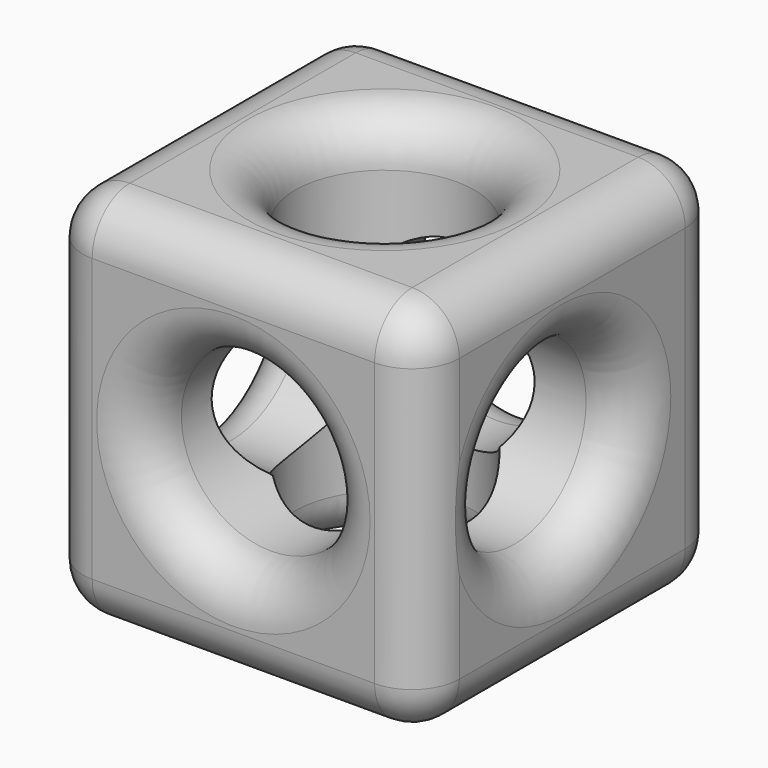
from build123d import *

# Parameters (mm, degrees)
F0_W         = 50.8
F0_H         = 50.8
F1_DEPTH     = 50.8
F3_D         = 24.20874
F5_D         = 24.20874
F7_D         = 24.20874
F8_T1_DEPTH  = 38.1
F8_T3_DEPTH  = 38.1
F8_T5_DEPTH  = 38.1
F8_S9_W      = 6.35
F8_S9_H      = 6.35
F8_T10_DEPTH = 6.35
F8_S15_W     = 6.35
F8_S15_H     = 6.35
F8_T16_DEPTH = 6.35
F8_S21_W     = 6.35
F8_S21_H     = 6.35
F8_T22_DEPTH = 6.35
F8_S27_W     = 6.35
F8_S27_H     = 6.35
F8_T28_DEPTH = 6.35
F8_S33_W     = 6.35
F8_S33_H     = 6.35
F8_T34_DEPTH = 6.35
F8_S39_W     = 6.35
F8_S39_H     = 6.35
F8_T40_DEPTH = 6.35
F8_S45_W     = 6.35
F8_S45_H     = 6.35
F8_T46_DEPTH = 6.35
F8_S51_W     = 6.35
F8_S51_H     = 6.35
F8_T52_DEPTH = 6.35


# Not quite as in the source:
# - a fillet or chamfer that OpenCascade refuses, or shapes differently, is made with other operations: its cross-section is extruded or revolved along the edge and cut away or added


with BuildPart() as f1:
    # F0 (on Front) → F1 (new body)
    with BuildSketch(Plane.XZ):
        Rectangle(F0_W, F0_H)
    extrude(amount=F1_DEPTH)

    # F3 (through all)
    with Locations(Plane.XZ.offset(50.8)):
        with Locations((0, 0)):
            Hole(F3_D / 2)

    # F5 (through all)
    with Locations(Plane.XY.offset(25.4)):
        with Locations((0, -25.266315788)):
            Hole(F5_D / 2)

    # F7 (through all)
    with Locations(Plane.YZ.offset(25.4)):
        with Locations((-27.2314734757, 0)):
            Hole(F7_D / 2)

    # F8: fillet of radius 6.35 on 18 edges, made by hand

    # F8_s2 → F8_t1 (cut)
    with BuildSketch(Plane.YZ.offset(-19.05)):
        with BuildLine():
            ThreePointArc((-50.8, 19.05), (-48.9401280605, 23.5401280605), (-44.45, 25.4))
            Line((-44.45, 25.4), (-50.8, 25.4))
            Line((-50.8, 25.4), (-50.8, 19.05))
        make_face()
        with BuildLine():
            ThreePointArc((0, 19.05), (-1.8598719395, 23.5401280605), (-6.35, 25.4))
            Line((-6.35, 25.4), (0, 25.4))
            Line((0, 25.4), (0, 19.05))
        make_face()
        with BuildLine():
            ThreePointArc((-44.45, -25.4), (-48.9401280605, -23.5401280605), (-50.8, -19.05))
            Line((-50.8, -19.05), (-50.8, -25.4))
            Line((-50.8, -25.4), (-44.45, -25.4))
        make_face()
        with BuildLine():
            ThreePointArc((-6.35, -25.4), (-1.8598719395, -23.5401280605), (0, -19.05))
            Line((0, -19.05), (0, -25.4))
            Line((0, -25.4), (-6.35, -25.4))
        make_face()
    extrude(amount=F8_T1_DEPTH, mode=Mode.SUBTRACT)

    # F8_s4 → F8_t3 (cut)
    with BuildSketch(Plane.XZ.offset(6.35)):
        with BuildLine():
            ThreePointArc((25.4, 19.05), (23.5401280605, 23.5401280605), (19.05, 25.4))
            Line((19.05, 25.4), (25.4, 25.4))
            Line((25.4, 25.4), (25.4, 19.05))
        make_face()
        with BuildLine():
            ThreePointArc((25.4, -19.05), (23.5401280605, -23.5401280605), (19.05, -25.4))
            Line((19.05, -25.4), (25.4, -25.4))
            Line((25.4, -25.4), (25.4, -19.05))
        make_face()
        with BuildLine():
            ThreePointArc((-19.05, 25.4), (-23.5401280605, 23.5401280605), (-25.4, 19.05))
            Line((-25.4, 19.05), (-25.4, 25.4))
            Line((-25.4, 25.4), (-19.05, 25.4))
        make_face()
        with BuildLine():
            ThreePointArc((-19.05, -25.4), (-23.5401280605, -23.5401280605), (-25.4, -19.05))
            Line((-25.4, -19.05), (-25.4, -25.4))
            Line((-25.4, -25.4), (-19.05, -25.4))
        make_face()
    extrude(amount=F8_T3_DEPTH, mode=Mode.SUBTRACT)

    # F8_s6 → F8_t5 (cut)
    with BuildSketch(Plane.XY.offset(-19.05)):
        with BuildLine():
            ThreePointArc((25.4, -44.45), (23.5401280605, -48.9401280605), (19.05, -50.8))
            Line((19.05, -50.8), (25.4, -50.8))
            Line((25.4, -50.8), (25.4, -44.45))
        make_face()
        with BuildLine():
            ThreePointArc((25.4, -6.35), (23.5401280605, -1.8598719395), (19.05, 0))
            Line((19.05, 0), (25.4, 0))
            Line((25.4, 0), (25.4, -6.35))
        make_face()
        with BuildLine():
            ThreePointArc((-19.05, -50.8), (-23.5401280605, -48.9401280605), (-25.4, -44.45))
            Line((-25.4, -44.45), (-25.4, -50.8))
            Line((-25.4, -50.8), (-19.05, -50.8))
        make_face()
        with BuildLine():
            ThreePointArc((-19.05, 0), (-23.5401280605, -1.8598719395), (-25.4, -6.35))
            Line((-25.4, -6.35), (-25.4, 0))
            Line((-25.4, 0), (-19.05, 0))
        make_face()
    extrude(amount=F8_T5_DEPTH, mode=Mode.SUBTRACT)


with BuildPart() as f8_tool8:
    # F8_s9 → F8_t10 (new body)
    with BuildSketch(Plane.YZ.offset(19.05)):
        with Locations((-47.625, 22.225)):
            Rectangle(F8_S9_W, F8_S9_H)
    extrude(amount=F8_T10_DEPTH)

    # F8_s11 → F8_t12 (revolve, cut)
    with BuildSketch(Plane(origin=(19.05, -44.45, 19.05), x_dir=(0, 0.7071067812, -0.7071067812), z_dir=(0, -0.7071067812, -0.7071067812))):
        with BuildLine():
            ThreePointArc((0, -6.35), (6.35, 0), (0, 6.35))
            Line((0, 6.35), (0, -6.35))
        make_face()
    revolve(axis=Axis((19.05, -44.45, 19.05), (1, 0, 0)), mode=Mode.SUBTRACT)


with BuildPart() as f1_1:
    add(f1.part)

    # F8_t7: cut F8_tool8
    add(f8_tool8.part, mode=Mode.SUBTRACT)


with BuildPart() as f8_tool14:
    # F8_s15 → F8_t16 (new body)
    with BuildSketch(Plane.XZ.offset(44.45)):
        with Locations((-22.225, 22.225)):
            Rectangle(F8_S15_W, F8_S15_H)
    extrude(amount=F8_T16_DEPTH)

    # F8_s17 → F8_t18 (revolve, cut)
    with BuildSketch(Plane(origin=(-19.05, -44.45, 19.05), x_dir=(0.7071067812, 0, -0.7071067812), z_dir=(-0.7071067812, 0, -0.7071067812))):
        with BuildLine():
            ThreePointArc((0, -6.35), (6.35, 0), (0, 6.35))
            Line((0, 6.35), (0, -6.35))
        make_face()
    revolve(axis=Axis((-19.05, -44.45, 19.05), (0, -1, 0)), mode=Mode.SUBTRACT)


with BuildPart() as f1_2:
    add(f1_1.part)

    # F8_t13: cut F8_tool14
    add(f8_tool14.part, mode=Mode.SUBTRACT)


with BuildPart() as f8_tool20:
    # F8_s21 → F8_t22 (new body)
    with BuildSketch(Plane.YZ.offset(19.05)):
        with Locations((-3.175, 22.225)):
            Rectangle(F8_S21_W, F8_S21_H)
    extrude(amount=F8_T22_DEPTH)

    # F8_s23 → F8_t24 (revolve, cut)
    with BuildSketch(Plane(origin=(19.05, -6.35, 19.05), x_dir=(0, -0.7071067812, -0.7071067812), z_dir=(0, -0.7071067812, 0.7071067812))):
        with BuildLine():
            ThreePointArc((0, -6.35), (6.35, 0), (0, 6.35))
            Line((0, 6.35), (0, -6.35))
        make_face()
    revolve(axis=Axis((19.05, -6.35, 19.05), (1, 0, 0)), mode=Mode.SUBTRACT)


with BuildPart() as f1_3:
    add(f1_2.part)

    # F8_t19: cut F8_tool20
    add(f8_tool20.part, mode=Mode.SUBTRACT)


with BuildPart() as f8_tool26:
    # F8_s27 → F8_t28 (new body)
    with BuildSketch(Plane.YZ.offset(19.05)):
        with Locations((-47.625, -22.225)):
            Rectangle(F8_S27_W, F8_S27_H)
    extrude(amount=F8_T28_DEPTH)

    # F8_s29 → F8_t30 (revolve, cut)
    with BuildSketch(Plane(origin=(19.05, -44.45, -19.05), x_dir=(0, 0.7071067812, 0.7071067812), z_dir=(0, 0.7071067812, -0.7071067812))):
        with BuildLine():
            ThreePointArc((0, -6.35), (6.35, 0), (0, 6.35))
            Line((0, 6.35), (0, -6.35))
        make_face()
    revolve(axis=Axis((19.05, -44.45, -19.05), (1, 0, 0)), mode=Mode.SUBTRACT)


with BuildPart() as f1_4:
    add(f1_3.part)

    # F8_t25: cut F8_tool26
    add(f8_tool26.part, mode=Mode.SUBTRACT)


with BuildPart() as f8_tool32:
    # F8_s33 → F8_t34 (new body)
    with BuildSketch(Plane.YZ.offset(19.05)):
        with Locations((-3.175, -22.225)):
            Rectangle(F8_S33_W, F8_S33_H)
    extrude(amount=F8_T34_DEPTH)

    # F8_s35 → F8_t36 (revolve, cut)
    with BuildSketch(Plane(origin=(19.05, -6.35, -19.05), x_dir=(0, -0.7071067812, 0.7071067812), z_dir=(0, 0.7071067812, 0.7071067812))):
        with BuildLine():
            ThreePointArc((0, -6.35), (6.35, 0), (0, 6.35))
            Line((0, 6.35), (0, -6.35))
        make_face()
    revolve(axis=Axis((19.05, -6.35, -19.05), (1, 0, 0)), mode=Mode.SUBTRACT)


with BuildPart() as f1_5:
    add(f1_4.part)

    # F8_t31: cut F8_tool32
    add(f8_tool32.part, mode=Mode.SUBTRACT)


with BuildPart() as f8_tool38:
    # F8_s39 → F8_t40 (new body)
    with BuildSketch(Plane.XZ.offset(6.35)):
        with Locations((-22.225, 22.225)):
            Rectangle(F8_S39_W, F8_S39_H)
    extrude(amount=-F8_T40_DEPTH)

    # F8_s41 → F8_t42 (revolve, cut)
    with BuildSketch(Plane(origin=(-19.05, -6.35, 19.05), x_dir=(0.7071067812, 0, -0.7071067812), z_dir=(0.7071067812, 0, 0.7071067812))):
        with BuildLine():
            ThreePointArc((0, -6.35), (6.35, 0), (0, 6.35))
            Line((0, 6.35), (0, -6.35))
        make_face()
    revolve(axis=Axis((-19.05, -6.35, 19.05), (0, 1, 0)), mode=Mode.SUBTRACT)


with BuildPart() as f1_6:
    add(f1_5.part)

    # F8_t37: cut F8_tool38
    add(f8_tool38.part, mode=Mode.SUBTRACT)


with BuildPart() as f8_tool44:
    # F8_s45 → F8_t46 (new body)
    with BuildSketch(Plane.XY.offset(-19.05)):
        with Locations((-22.225, -47.625)):
            Rectangle(F8_S45_W, F8_S45_H)
    extrude(amount=-F8_T46_DEPTH)

    # F8_s47 → F8_t48 (revolve, cut)
    with BuildSketch(Plane(origin=(-19.05, -44.45, -19.05), x_dir=(0.7071067812, 0.7071067812, 0), z_dir=(-0.7071067812, 0.7071067812, 0))):
        with BuildLine():
            ThreePointArc((0, -6.35), (6.35, 0), (0, 6.35))
            Line((0, 6.35), (0, -6.35))
        make_face()
    revolve(axis=Axis((-19.05, -44.45, -19.05), (0, 0, -1)), mode=Mode.SUBTRACT)


with BuildPart() as f1_7:
    add(f1_6.part)

    # F8_t43: cut F8_tool44
    add(f8_tool44.part, mode=Mode.SUBTRACT)


with BuildPart() as f8_tool50:
    # F8_s51 → F8_t52 (new body)
    with BuildSketch(Plane.XY.offset(-19.05)):
        with Locations((-22.225, -3.175)):
            Rectangle(F8_S51_W, F8_S51_H)
    extrude(amount=-F8_T52_DEPTH)

    # F8_s53 → F8_t54 (revolve, cut)
    with BuildSketch(Plane(origin=(-19.05, -6.35, -19.05), x_dir=(0.7071067812, -0.7071067812, 0), z_dir=(0.7071067812, 0.7071067812, 0))):
        with BuildLine():
            ThreePointArc((0, -6.35), (6.35, 0), (0, 6.35))
            Line((0, 6.35), (0, -6.35))
        make_face()
    revolve(axis=Axis((-19.05, -6.35, -19.05), (0, 0, -1)), mode=Mode.SUBTRACT)


with BuildPart() as f1_8:
    add(f1_7.part)

    # F8_t49: cut F8_tool50
    add(f8_tool50.part, mode=Mode.SUBTRACT)

    # F8_s55 → F8_t56 (revolve, cut)
    with BuildSketch(Plane.XY):
        with BuildLine():
            ThreePointArc((25.4, -8.7771034757), (23.5401280605, -13.2672315362), (19.05, -15.1271034757))
            Line((19.05, -15.1271034757), (25.4, -15.1271034757))
            Line((25.4, -15.1271034757), (25.4, -8.7771034757))
        make_face()
    revolve(axis=Axis((25.4, -27.2314734757, 0), (1, 0, 0)), mode=Mode.SUBTRACT)

    # F8_s57 → F8_t58 (revolve, cut)
    with BuildSketch(Plane.XZ.offset(25.266315788)):
        with BuildLine():
            ThreePointArc((18.45437, -25.4), (13.9642419395, -23.5401280605), (12.10437, -19.05))
            Line((12.10437, -19.05), (12.10437, -25.4))
            Line((12.10437, -25.4), (18.45437, -25.4))
        make_face()
    revolve(axis=Axis((0, -25.266315788, -25.4), (0, 0, 1)), mode=Mode.SUBTRACT)

    # F8_s59 → F8_t60 (revolve, cut)
    with BuildSketch(Plane.XY):
        with BuildLine():
            ThreePointArc((18.45437, 0), (13.9642419395, -1.8598719395), (12.10437, -6.35))
            Line((12.10437, -6.35), (12.10437, 0))
            Line((12.10437, 0), (18.45437, 0))
        make_face()
    revolve(axis=Axis((0, 0, 0), (0, -1, 0)), mode=Mode.SUBTRACT)

    # F8_s61 → F8_t62 (revolve, cut)
    with BuildSketch(Plane.XY):
        with BuildLine():
            ThreePointArc((18.45437, -50.8), (13.9642419395, -48.9401280605), (12.10437, -44.45))
            Line((12.10437, -44.45), (12.10437, -50.8))
            Line((12.10437, -50.8), (18.45437, -50.8))
        make_face()
    revolve(axis=Axis((0, -50.8, 0), (0, -1, 0)), mode=Mode.SUBTRACT)

    # F8_s63 → F8_t64 (revolve, cut)
    with BuildSketch(Plane.XZ.offset(25.266315788)):
        with BuildLine():
            ThreePointArc((18.45437, 25.4), (13.9642419395, 23.5401280605), (12.10437, 19.05))
            Line((12.10437, 19.05), (12.10437, 25.4))
            Line((12.10437, 25.4), (18.45437, 25.4))
        make_face()
    revolve(axis=Axis((0, -25.266315788, 25.4), (0, 0, 1)), mode=Mode.SUBTRACT)

    # F8_s65 → F8_t66 (revolve, cut)
    with BuildSketch(Plane.XY):
        with BuildLine():
            ThreePointArc((-25.4, -8.7771034757), (-23.5401280605, -13.2672315362), (-19.05, -15.1271034757))
            Line((-19.05, -15.1271034757), (-25.4, -15.1271034757))
            Line((-25.4, -15.1271034757), (-25.4, -8.7771034757))
        make_face()
    revolve(axis=Axis((-25.4, -27.2314734757, 0), (1, 0, 0)), mode=Mode.SUBTRACT)


solid = f1_8.part
